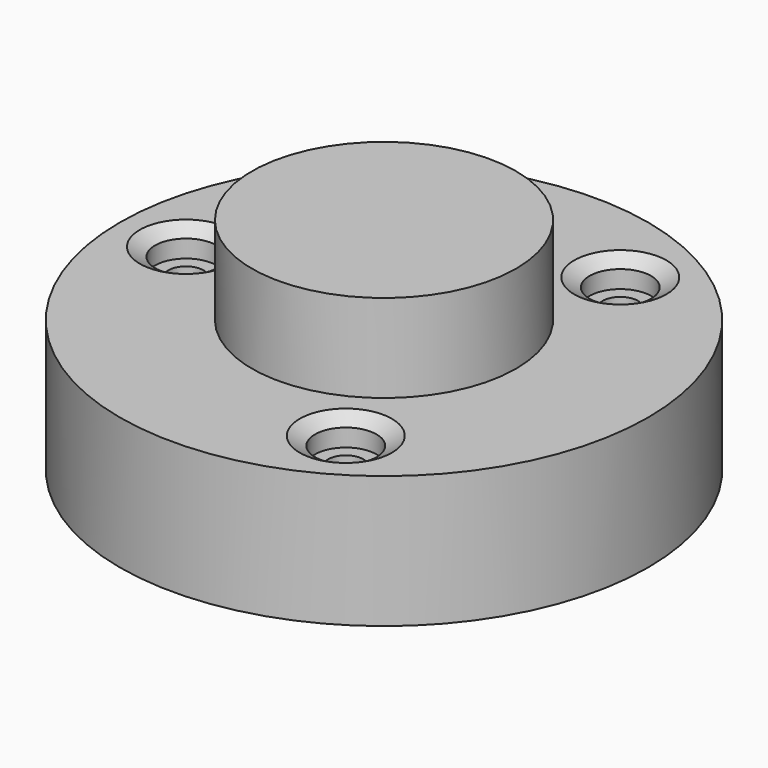
from build123d import *

# Parameters (mm, degrees)
F0_R       = 30
F0_R_2     = 3.5
F0_R_3     = 15
F1_DEPTH   = 15
F2_DEPTH   = 25
F0_R_4     = 2
F3_DEPTH   = 12
F4_SIZE2   = 1.7320508076
F4_SIZE    = 1
F4_2_SIZE2 = 1.7320508076
F4_2_SIZE  = 1
F4_3_SIZE2 = 1.7320508076
F4_3_SIZE  = 1


with BuildPart() as f1:
    # F0 (on Top) → F1 (new body)
    with BuildSketch(Plane.XY):
        Circle(F0_R)
        with Locations((11.25, -19.4855715851)):
            Circle(F0_R_2, mode=Mode.SUBTRACT)
        with Locations((-22.5, 0)):
            Circle(F0_R_2, mode=Mode.SUBTRACT)
        Circle(F0_R_3, mode=Mode.SUBTRACT)
        with Locations((11.25, 19.4855715851)):
            Circle(F0_R_2, mode=Mode.SUBTRACT)
    extrude(amount=F1_DEPTH)

    # F0 (on Top) → F2 (join)
    with BuildSketch(Plane.XY):
        Circle(F0_R_3)
    extrude(amount=F2_DEPTH)

    # F0 (on Top) → F3 (join)
    with BuildSketch(Plane.XY):
        with Locations((11.25, 19.4855715851)):
            Circle(F0_R_2)
        with Locations((11.25, 19.4855715851)):
            Circle(F0_R_4, mode=Mode.SUBTRACT)
        with Locations((11.25, -19.4855715851)):
            Circle(F0_R_2)
        with Locations((11.25, -19.4855715851)):
            Circle(F0_R_4, mode=Mode.SUBTRACT)
        with Locations((-22.5, 0)):
            Circle(F0_R_2)
        with Locations((-22.5, 0)):
            Circle(F0_R_4, mode=Mode.SUBTRACT)
    extrude(amount=F3_DEPTH)

    # F4
    f4_edges = [f1.edges().sort_by_distance(p)[0] for p in [
        (-26, 0, 15),
    ]]
    f4_side = f1.faces().sort_by_distance((-26, 0, 13.5))[0]
    chamfer(f4_edges, length=F4_SIZE, length2=F4_SIZE2, reference=f4_side)

    # F4#2
    f4_2_edges = [f1.edges().sort_by_distance(p)[0] for p in [
        (7.75, -19.485572, 15),
    ]]
    f4_2_side = f1.faces().sort_by_distance((7.75, -19.485572, 13.5))[0]
    chamfer(f4_2_edges, length=F4_2_SIZE, length2=F4_2_SIZE2, reference=f4_2_side)

    # F4#3
    f4_3_edges = [f1.edges().sort_by_distance(p)[0] for p in [
        (7.75, 19.485572, 15),
    ]]
    f4_3_side = f1.faces().sort_by_distance((7.75, 19.485572, 13.5))[0]
    chamfer(f4_3_edges, length=F4_3_SIZE, length2=F4_3_SIZE2, reference=f4_3_side)


solid = f1.part
